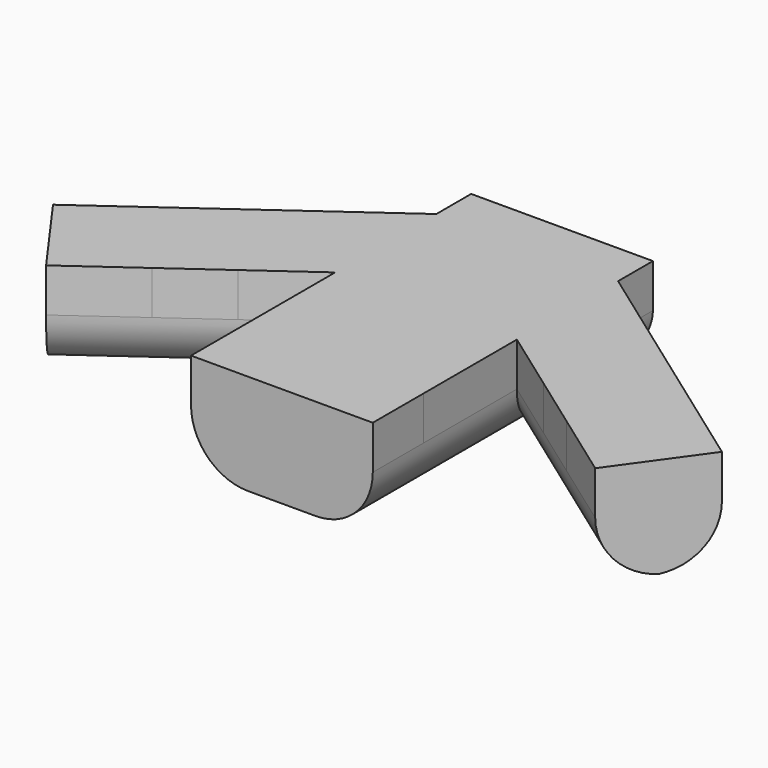
from build123d import *

# Parameters (mm, degrees)
F0_W          = 10.8273038641
F0_H          = 3.767536847
F0_H_2        = 3.7791659124
F0_H_3        = 3.1744926237
F1_DEPTH      = 6
F2_T1_DEPTH   = 27.8273038641
F2_T6_DEPTH   = 34.8580118286
F2_T11_DEPTH  = 30.4667466587
F2_T16_DEPTH  = 27.7328249142
F2_T21_DEPTH  = 27.7328249142
F2_T26_DEPTH  = 27.7328249142
F2_T31_DEPTH  = 27.7328249142
F2_T36_DEPTH  = 30.4667466587
F2_T41_DEPTH  = 34.8580118286
F2_T46_DEPTH  = 19.5930984205
F2_T51_DEPTH  = 19.5930984205
F2_T56_DEPTH  = 19.5930984205
F2_T61_DEPTH  = 19.5930984205
F2_T67_DEPTH  = 34.8580118286
F2_T71_DEPTH  = 19.5930984205
F2_T79_DEPTH  = 27.7328249142
F2_T84_DEPTH  = 30.4667466587
F2_T91_DEPTH  = 30.4667466587
F2_T95_DEPTH  = 27.7328249142
F2_T103_DEPTH = 19.5930984205
F2_T108_DEPTH = 34.8580118286


# Not quite as in the source:
# - a fillet or chamfer that OpenCascade refuses, or shapes differently, is made with other operations: its cross-section is extruded or revolved along the edge and cut away or added


with BuildPart() as f1:
    # F0 (on Top) → F1 (new body)
    with BuildSketch(Plane.XY):
        Polygon((-16.3571660357, -7.848105799), (-12.3521852931, -4.9759467929), (-15.9206694666, 0), (-19.9256502092, -2.8721590061), align=None)
        Polygon((-12.3521852931, -4.9759467929), (-9.1011668972, -2.644489449), (-12.6696510706, 2.331457344), (-15.9206694666, 0), align=None)
        Polygon((-9.1011668972, -2.644489449), (-5.413651932, 0), (-8.7160122578, 5.1667966509), (-12.6696510706, 2.331457344), align=None)
        Polygon((-8.7160122578, 5.1667966509), (-5.413651932, 0), (-5.413651932, 3.767536847), (-5.413651932, 7.535073694), align=None)
        Polygon((-5.413651932, 7.535073694), (-5.413651932, 3.767536847), (5.413651932, 3.767536847), (5.413651932, 7.535073694), (0, 7.535073694), align=None)
        Polygon((-5.413651932, 10.1281721145), (-5.413651932, 7.535073694), (0, 7.535073694), (5.413651932, 7.535073694), (5.413651932, 10.1281721145), (0, 10.1281721145), align=None)
        Polygon((5.413651932, 3.767536847), (5.413651932, 0), (8.7160122578, 5.1667966509), (5.413651932, 7.535073694), align=None)
        Polygon((8.7160122578, 5.1667966509), (5.413651932, 0), (9.1011668972, -2.644489449), (12.6696510706, 2.331457344), align=None)
        Polygon((12.6696510706, 2.331457344), (9.1011668972, -2.644489449), (12.3521852931, -4.9759467929), (15.9206694666, 0), align=None)
        Polygon((15.9206694666, 0), (12.3521852931, -4.9759467929), (16.3571660357, -7.848105799), (19.9256502092, -2.8721590061), align=None)
        with Locations((0, 1.8837684235)):
            Rectangle(F0_W, F0_H)
        with Locations((0, -5.0640755799)):
            Rectangle(F0_W, F0_H_2)
        with Locations((0, -1.5872463118)):
            Rectangle(F0_W, F0_H_3)
        Polygon((5.413651932, -6.9536585361), (-5.413651932, -6.9536585361), (-5.413651932, -10.7328249142), (0, -10.7328249142), (5.413651932, -10.7328249142), align=None)
    extrude(amount=F1_DEPTH)

    # F2: fillet of radius 3.4 on 9 edges, made by hand

    # F2_s2 → F2_t1 (cut)
    with BuildSketch(Plane.YZ.offset(-13.913651932)):
        with BuildLine():
            ThreePointArc((10.1281721145, 3.4), (9.1323351705, 0.995836944), (6.7281721145, 0))
            Line((6.7281721145, 0), (10.1281721145, 0))
            Line((10.1281721145, 0), (10.1281721145, 3.4))
        make_face()
    extrude(amount=F2_T1_DEPTH, mode=Mode.SUBTRACT)


with BuildPart() as f2_tool4:
    # F2_s5 → F2_t6 (new body)
    with BuildSketch(Plane(origin=(21.4259097927, -15.365522016, 0), x_dir=(0, 0, 1), z_dir=(-0.8126323589, 0.5827766719, 0))):
        with BuildLine():
            ThreePointArc((3.4, 9.278194766), (0.995836944, 8.2823578221), (0, 5.878194766))
            Line((0, 5.878194766), (0, 9.278194766))
            Line((0, 9.278194766), (3.4, 9.278194766))
        make_face()
    extrude(amount=F2_T6_DEPTH)

    split(bisect_by=Plane.YZ.offset(5.413651932), keep=Keep.TOP)


with BuildPart() as f1_1:
    add(f1.part)

    # F2_t3: cut F2_tool4
    add(f2_tool4.part, mode=Mode.SUBTRACT)


with BuildPart() as f2_tool9:
    # F2_s10 → F2_t11 (new body)
    with BuildSketch(Plane(origin=(-3.3323544119, 2.3897872052, 0), x_dir=(0, 0, 1), z_dir=(0.8126323589, -0.5827766719, 0))):
        with BuildLine():
            ThreePointArc((3.4, -3.1549500557), (0.995836944, -4.1507869997), (0, -6.5549500557))
            Line((0, -6.5549500557), (0, -3.1549500557))
            Line((0, -3.1549500557), (3.4, -3.1549500557))
        make_face()
    extrude(amount=F2_T11_DEPTH)

    split(bisect_by=Plane.YZ.offset(5.413651932), keep=Keep.TOP)


with BuildPart() as f1_2:
    add(f1_1.part)

    # F2_t8: cut F2_tool9
    add(f2_tool9.part, mode=Mode.SUBTRACT)


with BuildPart() as f2_tool14:
    # F2_s15 → F2_t16 (new body)
    with BuildSketch(Plane.XZ.offset(19.2328249142)):
        with BuildLine():
            ThreePointArc((5.413651932, 3.4), (4.4178149881, 0.995836944), (2.013651932, 0))
            Line((2.013651932, 0), (5.413651932, 0))
            Line((5.413651932, 0), (5.413651932, 3.4))
        make_face()
    extrude(amount=-F2_T16_DEPTH)

    split(bisect_by=Plane(origin=(1.8386312935, 2.5638145059, 0), x_dir=(0, 0, 1), z_dir=(-0.5827766719, -0.8126323589, 0)), keep=Keep.TOP)


with BuildPart() as f1_3:
    add(f1_2.part)

    # F2_t13: cut F2_tool14
    add(f2_tool14.part, mode=Mode.SUBTRACT)


with BuildPart() as f2_tool19:
    # F2_s20 → F2_t21 (new body)
    with BuildSketch(Plane.XZ.offset(19.2328249142)):
        with BuildLine():
            ThreePointArc((5.413651932, 3.4), (4.4178149881, 0.995836944), (2.013651932, 0))
            Line((2.013651932, 0), (5.413651932, 0))
            Line((5.413651932, 0), (5.413651932, 3.4))
        make_face()
    extrude(amount=-F2_T21_DEPTH)

    split(bisect_by=Plane(origin=(5.4071154669, 7.5397612989, 0), x_dir=(0, 0, 1), z_dir=(0.5827766719, 0.8126323589, 0)), keep=Keep.TOP)


with BuildPart() as f1_4:
    add(f1_3.part)

    # F2_t18: cut F2_tool19
    add(f2_tool19.part, mode=Mode.SUBTRACT)


with BuildPart() as f2_tool24:
    # F2_s25 → F2_t26 (new body)
    with BuildSketch(Plane.XZ.offset(-8.5)):
        with BuildLine():
            ThreePointArc((-5.413651932, 3.4), (-4.4178149881, 0.995836944), (-2.013651932, 0))
            Line((-2.013651932, 0), (-5.413651932, 0))
            Line((-5.413651932, 0), (-5.413651932, 3.4))
        make_face()
    extrude(amount=F2_T26_DEPTH)

    split(bisect_by=Plane(origin=(-5.4071154669, 7.5397612989, 0), x_dir=(0, 0, 1), z_dir=(-0.5827766719, 0.8126323589, 0)), keep=Keep.TOP)


with BuildPart() as f1_5:
    add(f1_4.part)

    # F2_t23: cut F2_tool24
    add(f2_tool24.part, mode=Mode.SUBTRACT)


with BuildPart() as f2_tool29:
    # F2_s30 → F2_t31 (new body)
    with BuildSketch(Plane.XZ.offset(-8.5)):
        with BuildLine():
            ThreePointArc((-5.413651932, 3.4), (-4.4178149881, 0.995836944), (-2.013651932, 0))
            Line((-2.013651932, 0), (-5.413651932, 0))
            Line((-5.413651932, 0), (-5.413651932, 3.4))
        make_face()
    extrude(amount=F2_T31_DEPTH)

    split(bisect_by=Plane(origin=(-1.8386312935, 2.5638145059, 0), x_dir=(0, 0, 1), z_dir=(0.5827766719, -0.8126323589, 0)), keep=Keep.TOP)


with BuildPart() as f1_6:
    add(f1_5.part)

    # F2_t28: cut F2_tool29
    add(f2_tool29.part, mode=Mode.SUBTRACT)


with BuildPart() as f2_tool34:
    # F2_s35 → F2_t36 (new body)
    with BuildSketch(Plane(origin=(-21.4259097927, -15.365522016, 0), x_dir=(0, 0, 1), z_dir=(0.8126323589, 0.5827766719, 0))):
        with BuildLine():
            ThreePointArc((3.4, -3.1549500557), (0.995836944, -4.1507869997), (0, -6.5549500557))
            Line((0, -6.5549500557), (0, -3.1549500557))
            Line((0, -3.1549500557), (3.4, -3.1549500557))
        make_face()
    extrude(amount=F2_T36_DEPTH)

    split(bisect_by=Plane.YZ.offset(-5.413651932), keep=Keep.BOTTOM)


with BuildPart() as f1_7:
    add(f1_6.part)

    # F2_t33: cut F2_tool34
    add(f2_tool34.part, mode=Mode.SUBTRACT)


with BuildPart() as f2_tool39:
    # F2_s40 → F2_t41 (new body)
    with BuildSketch(Plane(origin=(6.9008385854, 4.9489141062, 0), x_dir=(0, 0, 1), z_dir=(-0.8126323589, -0.5827766719, 0))):
        with BuildLine():
            ThreePointArc((3.4, 9.278194766), (0.995836944, 8.2823578221), (0, 5.878194766))
            Line((0, 5.878194766), (0, 9.278194766))
            Line((0, 9.278194766), (3.4, 9.278194766))
        make_face()
    extrude(amount=F2_T41_DEPTH)

    split(bisect_by=Plane.YZ.offset(-5.413651932), keep=Keep.BOTTOM)


with BuildPart() as f1_8:
    add(f1_7.part)

    # F2_t38: cut F2_tool39
    add(f2_tool39.part, mode=Mode.SUBTRACT)


with BuildPart() as f2_tool44:
    # F2_s45 → F2_t46 (new body)
    with BuildSketch(Plane.XZ.offset(0.964926306)):
        with BuildLine():
            ThreePointArc((5.413651932, 3.4), (4.4178149881, 0.995836944), (2.013651932, 0))
            Line((2.013651932, 0), (5.413651932, 0))
            Line((5.413651932, 0), (5.413651932, 3.4))
        make_face()
    extrude(amount=-F2_T46_DEPTH)

    split(bisect_by=Plane(origin=(1.8386312935, 2.5638145059, 0), x_dir=(0, 0, 1), z_dir=(-0.5827766719, -0.8126323589, 0)), keep=Keep.TOP)


with BuildPart() as f1_9:
    add(f1_8.part)

    # F2_t43: cut F2_tool44
    add(f2_tool44.part, mode=Mode.SUBTRACT)


with BuildPart() as f2_tool49:
    # F2_s50 → F2_t51 (new body)
    with BuildSketch(Plane.XZ.offset(0.964926306)):
        with BuildLine():
            ThreePointArc((5.413651932, 3.4), (4.4178149881, 0.995836944), (2.013651932, 0))
            Line((2.013651932, 0), (5.413651932, 0))
            Line((5.413651932, 0), (5.413651932, 3.4))
        make_face()
    extrude(amount=-F2_T51_DEPTH)

    split(bisect_by=Plane(origin=(5.4071154669, 7.5397612989, 0), x_dir=(0, 0, 1), z_dir=(0.5827766719, 0.8126323589, 0)), keep=Keep.TOP)


with BuildPart() as f1_10:
    add(f1_9.part)

    # F2_t48: cut F2_tool49
    add(f2_tool49.part, mode=Mode.SUBTRACT)


with BuildPart() as f2_tool54:
    # F2_s55 → F2_t56 (new body)
    with BuildSketch(Plane.XZ.offset(-18.6281721145)):
        with BuildLine():
            ThreePointArc((-5.413651932, 3.4), (-4.4178149881, 0.995836944), (-2.013651932, 0))
            Line((-2.013651932, 0), (-5.413651932, 0))
            Line((-5.413651932, 0), (-5.413651932, 3.4))
        make_face()
    extrude(amount=F2_T56_DEPTH)

    split(bisect_by=Plane(origin=(-5.4071154669, 7.5397612989, 0), x_dir=(0, 0, 1), z_dir=(-0.5827766719, 0.8126323589, 0)), keep=Keep.TOP)


with BuildPart() as f1_11:
    add(f1_10.part)

    # F2_t53: cut F2_tool54
    add(f2_tool54.part, mode=Mode.SUBTRACT)


with BuildPart() as f2_tool59:
    # F2_s60 → F2_t61 (new body)
    with BuildSketch(Plane.XZ.offset(-18.6281721145)):
        with BuildLine():
            ThreePointArc((-5.413651932, 3.4), (-4.4178149881, 0.995836944), (-2.013651932, 0))
            Line((-2.013651932, 0), (-5.413651932, 0))
            Line((-5.413651932, 0), (-5.413651932, 3.4))
        make_face()
    extrude(amount=F2_T61_DEPTH)

    split(bisect_by=Plane(origin=(-1.8386312935, 2.5638145059, 0), x_dir=(0, 0, 1), z_dir=(0.5827766719, -0.8126323589, 0)), keep=Keep.TOP)


with BuildPart() as f1_12:
    add(f1_11.part)

    # F2_t58: cut F2_tool59
    add(f2_tool59.part, mode=Mode.SUBTRACT)


with BuildPart() as f2_tool65:
    # F2_s66 → F2_t67 (new body)
    with BuildSketch(Plane(origin=(21.4259097927, -15.365522016, 0), x_dir=(0, 0, 1), z_dir=(-0.8126323589, 0.5827766719, 0))):
        with BuildLine():
            ThreePointArc((3.4, 9.278194766), (0.995836944, 8.2823578221), (0, 5.878194766))
            Line((0, 5.878194766), (0, 9.278194766))
            Line((0, 9.278194766), (3.4, 9.278194766))
        make_face()
    extrude(amount=F2_T67_DEPTH)

    split(bisect_by=Plane.YZ.offset(5.413651932), keep=Keep.BOTTOM)


with BuildPart() as f2_tool69:
    # F2_s70 → F2_t71 (new body)
    with BuildSketch(Plane.XZ.offset(0.964926306)):
        with BuildLine():
            ThreePointArc((5.413651932, 3.4), (4.4178149881, 0.995836944), (2.013651932, 0))
            Line((2.013651932, 0), (5.413651932, 0))
            Line((5.413651932, 0), (5.413651932, 3.4))
        make_face()
    extrude(amount=-F2_T71_DEPTH)

    split(bisect_by=Plane(origin=(1.8386312935, 2.5638145059, 0), x_dir=(0, 0, 1), z_dir=(0.5827766719, 0.8126323589, 0)), keep=Keep.TOP)

    split(bisect_by=Plane(origin=(5.4071154669, 7.5397612989, 0), x_dir=(0, 0, 1), z_dir=(-0.5827766719, -0.8126323589, 0)), keep=Keep.TOP)


with BuildPart() as f2_tool65_1:
    add(f2_tool65.part)

    # F2_t74: intersect F2_tool69
    add(f2_tool69.part, mode=Mode.INTERSECT)


with BuildPart() as f1_13:
    add(f1_12.part)

    # F2_t63: cut F2_tool65
    add(f2_tool65_1.part, mode=Mode.SUBTRACT)


with BuildPart() as f2_tool77:
    # F2_s78 → F2_t79 (new body)
    with BuildSketch(Plane.XZ.offset(19.2328249142)):
        with BuildLine():
            ThreePointArc((5.413651932, 3.4), (4.4178149881, 0.995836944), (2.013651932, 0))
            Line((2.013651932, 0), (5.413651932, 0))
            Line((5.413651932, 0), (5.413651932, 3.4))
        make_face()
    extrude(amount=-F2_T79_DEPTH)

    split(bisect_by=Plane(origin=(1.8386312935, 2.5638145059, 0), x_dir=(0, 0, 1), z_dir=(0.5827766719, 0.8126323589, 0)), keep=Keep.TOP)

    split(bisect_by=Plane(origin=(5.4071154669, 7.5397612989, 0), x_dir=(0, 0, 1), z_dir=(-0.5827766719, -0.8126323589, 0)), keep=Keep.TOP)


with BuildPart() as f2_tool82:
    # F2_s83 → F2_t84 (new body)
    with BuildSketch(Plane(origin=(-3.3323544119, 2.3897872052, 0), x_dir=(0, 0, 1), z_dir=(0.8126323589, -0.5827766719, 0))):
        with BuildLine():
            ThreePointArc((3.4, -3.1549500557), (0.995836944, -4.1507869997), (0, -6.5549500557))
            Line((0, -6.5549500557), (0, -3.1549500557))
            Line((0, -3.1549500557), (3.4, -3.1549500557))
        make_face()
    extrude(amount=F2_T84_DEPTH)

    split(bisect_by=Plane.YZ.offset(5.413651932), keep=Keep.BOTTOM)


with BuildPart() as f2_tool77_1:
    add(f2_tool77.part)

    # F2_t86: intersect F2_tool82
    add(f2_tool82.part, mode=Mode.INTERSECT)


with BuildPart() as f1_14:
    add(f1_13.part)

    # F2_t75: cut F2_tool77
    add(f2_tool77_1.part, mode=Mode.SUBTRACT)


with BuildPart() as f2_tool89:
    # F2_s90 → F2_t91 (new body)
    with BuildSketch(Plane(origin=(-21.4259097927, -15.365522016, 0), x_dir=(0, 0, 1), z_dir=(0.8126323589, 0.5827766719, 0))):
        with BuildLine():
            ThreePointArc((3.4, -3.1549500557), (0.995836944, -4.1507869997), (0, -6.5549500557))
            Line((0, -6.5549500557), (0, -3.1549500557))
            Line((0, -3.1549500557), (3.4, -3.1549500557))
        make_face()
    extrude(amount=F2_T91_DEPTH)

    split(bisect_by=Plane.YZ.offset(-5.413651932), keep=Keep.TOP)


with BuildPart() as f2_tool93:
    # F2_s94 → F2_t95 (new body)
    with BuildSketch(Plane.XZ.offset(-8.5)):
        with BuildLine():
            ThreePointArc((-5.413651932, 3.4), (-4.4178149881, 0.995836944), (-2.013651932, 0))
            Line((-2.013651932, 0), (-5.413651932, 0))
            Line((-5.413651932, 0), (-5.413651932, 3.4))
        make_face()
    extrude(amount=F2_T95_DEPTH)

    split(bisect_by=Plane(origin=(-1.8386312935, 2.5638145059, 0), x_dir=(0, 0, 1), z_dir=(-0.5827766719, 0.8126323589, 0)), keep=Keep.TOP)

    split(bisect_by=Plane(origin=(-5.4071154669, 7.5397612989, 0), x_dir=(0, 0, 1), z_dir=(0.5827766719, -0.8126323589, 0)), keep=Keep.TOP)


with BuildPart() as f2_tool89_1:
    add(f2_tool89.part)

    # F2_t98: intersect F2_tool93
    add(f2_tool93.part, mode=Mode.INTERSECT)


with BuildPart() as f1_15:
    add(f1_14.part)

    # F2_t87: cut F2_tool89
    add(f2_tool89_1.part, mode=Mode.SUBTRACT)


with BuildPart() as f2_tool101:
    # F2_s102 → F2_t103 (new body)
    with BuildSketch(Plane.XZ.offset(-18.6281721145)):
        with BuildLine():
            ThreePointArc((-5.413651932, 3.4), (-4.4178149881, 0.995836944), (-2.013651932, 0))
            Line((-2.013651932, 0), (-5.413651932, 0))
            Line((-5.413651932, 0), (-5.413651932, 3.4))
        make_face()
    extrude(amount=F2_T103_DEPTH)

    split(bisect_by=Plane(origin=(-1.8386312935, 2.5638145059, 0), x_dir=(0, 0, 1), z_dir=(-0.5827766719, 0.8126323589, 0)), keep=Keep.TOP)

    split(bisect_by=Plane(origin=(-5.4071154669, 7.5397612989, 0), x_dir=(0, 0, 1), z_dir=(0.5827766719, -0.8126323589, 0)), keep=Keep.TOP)


with BuildPart() as f2_tool106:
    # F2_s107 → F2_t108 (new body)
    with BuildSketch(Plane(origin=(6.9008385854, 4.9489141062, 0), x_dir=(0, 0, 1), z_dir=(-0.8126323589, -0.5827766719, 0))):
        with BuildLine():
            ThreePointArc((3.4, 9.278194766), (0.995836944, 8.2823578221), (0, 5.878194766))
            Line((0, 5.878194766), (0, 9.278194766))
            Line((0, 9.278194766), (3.4, 9.278194766))
        make_face()
    extrude(amount=F2_T108_DEPTH)

    split(bisect_by=Plane.YZ.offset(-5.413651932), keep=Keep.TOP)


with BuildPart() as f2_tool101_1:
    add(f2_tool101.part)

    # F2_t110: intersect F2_tool106
    add(f2_tool106.part, mode=Mode.INTERSECT)


with BuildPart() as f1_16:
    add(f1_15.part)

    # F2_t99: cut F2_tool101
    add(f2_tool101_1.part, mode=Mode.SUBTRACT)


solid = f1_16.part
